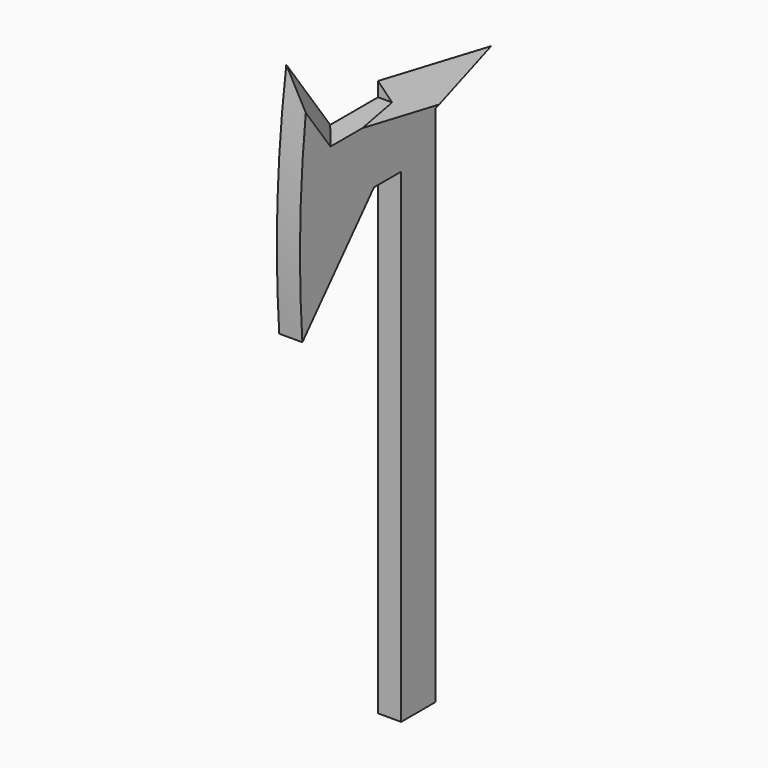
from build123d import *

# Parameters (mm, degrees)
F1_DEPTH    = 2.54
F2_T4_DEPTH = 40.6971516331
F3_T4_DEPTH = 48.3394519199
F4_T4_DEPTH = 63.1242461628


# Not quite as in the source:
# - a fillet or chamfer that OpenCascade refuses, or shapes differently, is made with other operations: its cross-section is extruded or revolved along the edge and cut away or added


with BuildPart() as f1:
    # F0 (on Right) → F1 (new body)
    with BuildSketch(Plane.YZ):
        Polygon((-0.3011617849, 0), (-4.707176704, 0), (-4.707176704, -3.2687797211), (-4.707176704, -9.6434028819), (-4.707176704, -62.8868843283), (0, -62.8868843283), (0, -10.7670552097), align=None)
        with BuildLine():
            Line((-4.707176704, -9.6434028819), (-4.707176704, -3.2687797211))
            Line((-4.707176704, -3.2687797211), (-8.1328889355, -3.2687797211))
            Line((-8.1328889355, -3.2687797211), (-16.7150776833, 8.5039641708))
            ThreePointArc((-16.7150776833, 8.5039641708), (-18.448774527, -6.0153747507), (-18.2778015733, -20.6368546933))
            Line((-18.2778015733, -20.6368546933), (-8.4392093122, -9.6434028819))
            Line((-8.4392093122, -9.6434028819), (-4.707176704, -9.6434028819))
        make_face()
        Polygon((0, 0), (-0.3011617849, 0), (0, -10.7670552097), (21.1573056877, -4.0066023357), align=None)
    extrude(amount=F1_DEPTH)

    # F2: chamfer of 5.08 on 1 edges, made by hand


with BuildPart() as f2_tool2:
    # F2_s3 → F2_t4 (new body)
    with BuildSketch(Plane(origin=(0, 6.4295894432, -8.8198840726), x_dir=(1, 0, 0), z_dir=(0, -0.5890778812, 0.8080762649))):
        Polygon((-2.54, -8.497560346), (2.54, -13.577560346), (2.54, -8.497560346), align=None)
    extrude(amount=F2_T4_DEPTH)

    split(bisect_by=Plane.XY.offset(-3.2687797211), keep=Keep.TOP)


with BuildPart() as f1_1:
    add(f1.part)

    # F2_t1: cut F2_tool2
    add(f2_tool2.part, mode=Mode.SUBTRACT)

    # F3: chamfer of 5.08 on 1 edges, made by hand


with BuildPart() as f3_tool2:
    # F3_s3 → F3_t4 (new body)
    with BuildSketch(Plane(origin=(0, -15.5659961488, -4.9738461482), x_dir=(1, 0, 0), z_dir=(0, 0.9525532472, 0.3043719948))):
        Polygon((2.54, 5.1761934028), (-2.54, 10.2561934028), (2.54, 10.2561934028), align=None)
    extrude(amount=F3_T4_DEPTH)

    split(bisect_by=Plane.XZ, keep=Keep.BOTTOM)


with BuildPart() as f1_2:
    add(f1_1.part)

    # F3_t1: cut F3_tool2
    add(f3_tool2.part, mode=Mode.SUBTRACT)

    # F4: chamfer of 5.08 on 1 edges, made by hand


with BuildPart() as f4_tool2:
    # F4_s3 → F4_t4 (new body)
    with BuildSketch(Plane(origin=(0, 23.513886354, -4.4528728458), x_dir=(1, 0, 0), z_dir=(0, -0.9825374139, 0.1860651236))):
        Polygon((2.54, -5.08), (-2.54, 0), (2.54, 0), align=None)
    extrude(amount=F4_T4_DEPTH)

    split(bisect_by=Plane(origin=(-5.518780173, -4.4595952689, -3.2509913312), x_dir=(-0.6285178248, 0.7777951812, 0), z_dir=(0.7071067812, 0.5713962066, 0.4165409645)), keep=Keep.TOP)


with BuildPart() as f1_3:
    add(f1_2.part)

    # F4_t1: cut F4_tool2
    add(f4_tool2.part, mode=Mode.SUBTRACT)


solid = f1_3.part
